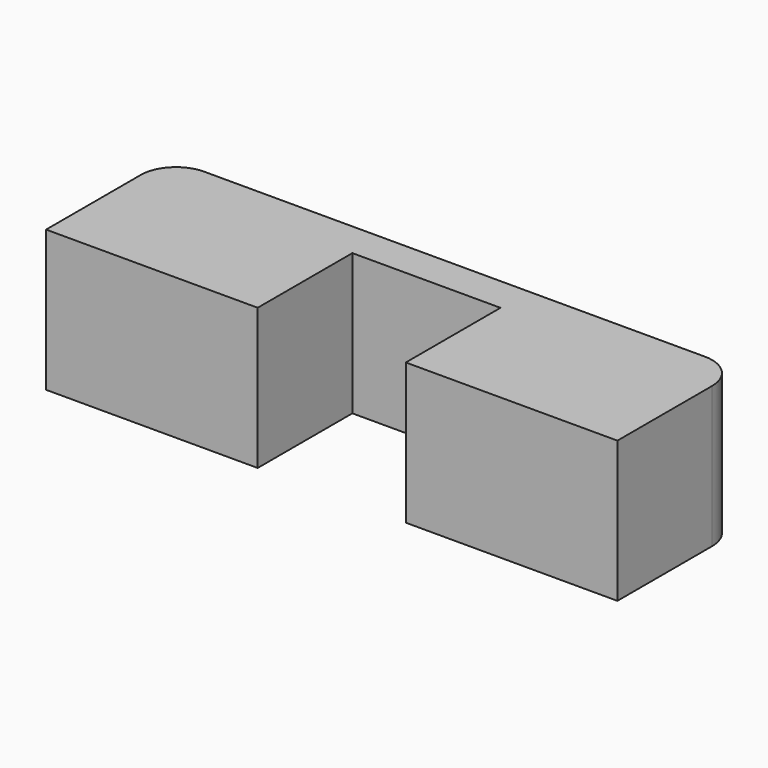
from build123d import *

# Parameters (mm, degrees)
F0_W     = 63.5
F0_H     = 12.7
F0_W_2   = 76.2
F0_H_2   = 25.4
F0_W_3   = 53.3399905968
F0_W_4   = 63.5000094032
F1_DEPTH = 50.8


# Not quite as in the source:
# - ends of sketch curves that miss each other by under 0.0002 mm in the source are joined


with BuildPart() as f1:
    # F0 (on Top) → F1 (new body)
    with BuildSketch(Plane.XY):
        with Locations((-58.4199952984, 21.9910541385)):
            Rectangle(F0_W, F0_H)
        with BuildLine():
            Line((-102.8699952984, 15.6410541385), (-102.8699952984, -1.5747001893))
            Line((-102.8699952984, -1.5747001893), (-26.6699952984, -1.5747001893))
            Line((-26.6699952984, -1.5747001893), (-26.6699952984, 15.6410541385))
            Line((-26.6699952984, 15.6410541385), (-90.1699952984, 15.6410541385))
            Line((-90.1699952984, 15.6410541385), (-90.1699952984, 28.3410541385))
            ThreePointArc((-90.1699952984, 28.3410541385), (-99.1502514195, 24.6213102596), (-102.8699952984, 15.6410541385))
        make_face()
        with Locations((-64.7699952984, -14.2747001893)):
            Rectangle(F0_W_2, F0_H_2)
        with Locations((0, 21.9910541385)):
            Rectangle(F0_W_3, F0_H)
        with Locations((58.42, 21.9910541385)):
            Rectangle(F0_W_4, F0_H)
        with BuildLine():
            Line((90.1700047016, 15.6410541385), (26.6699952984, 15.6410541385))
            Line((26.6699952984, 15.6410541385), (26.6699952984, -1.5747001893))
            Line((26.6699952984, -1.5747001893), (102.8699952984, -1.5747001893))
            Line((102.8699952984, -1.5747001893), (102.8699952984, 15.6410541385))
            ThreePointArc((102.8699952984, 15.6410541385), (99.1502514195, 24.6213102596), (90.1699952984, 28.3410541385))
            Line((90.1699952984, 28.3410541385), (90.1700047016, 15.6410541385))
        make_face()
        with Locations((64.7699952984, -14.2747001893)):
            Rectangle(F0_W_2, F0_H_2)
    extrude(amount=F1_DEPTH)


solid = f1.part
